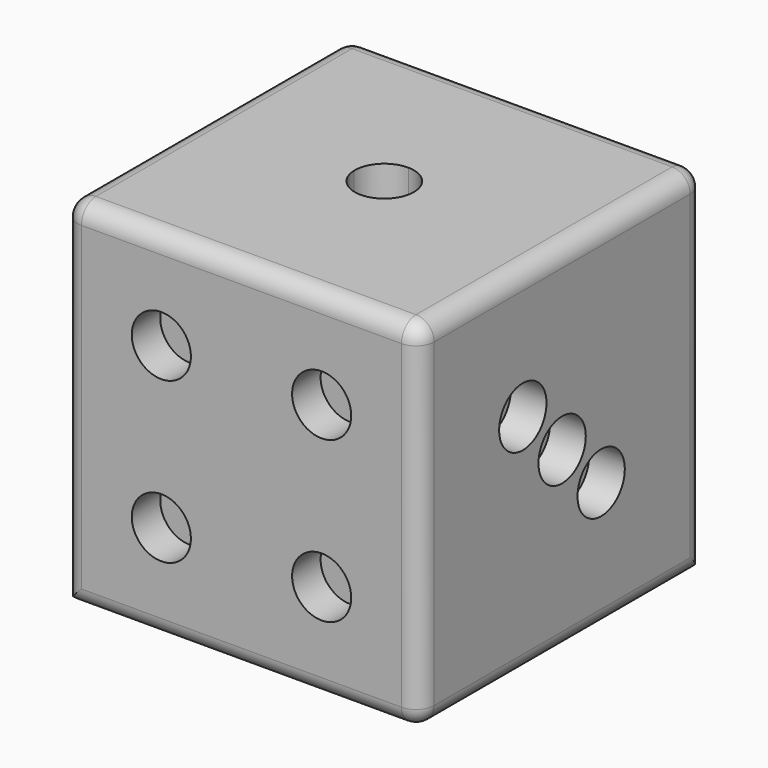
from build123d import *

# Parameters (mm, degrees)
F0_W         = 100
F0_H         = 100
F1_DEPTH     = 100
F2_R         = 5.08
F3_R         = 5.08
F4_T1_DEPTH  = 120.32
F4_T3_DEPTH  = 120.32
F5_T1_DEPTH  = 89.84
F5_S5_W      = 5.08
F5_S5_H      = 5.08
F5_T6_DEPTH  = 5.08
F5_S11_W     = 5.08
F5_S11_H     = 5.08
F5_T12_DEPTH = 5.08
F8_DEPTH     = 10
F10_R        = 8.3
F11_DEPTH    = 10
F12_R        = 8.3
F13_DEPTH    = 10
F9_R         = 8.3
F14_DEPTH    = 10
F15_R        = 8.3
F16_DEPTH    = 10
F17_R        = 8.3
F18_DEPTH    = 10


# Not quite as in the source:
# - a fillet or chamfer that OpenCascade refuses, or shapes differently, is made with other operations: its cross-section is extruded or revolved along the edge and cut away or added


with BuildPart() as f1:
    # F0 (on Top) → F1 (new body)
    with BuildSketch(Plane.XY):
        with Locations((-11.9530703868, 12.5334430486)):
            Rectangle(F0_W, F0_H)
    extrude(amount=F1_DEPTH)

    # F2
    f2_edges = [f1.edges().sort_by_distance(p)[0] for p in [
        (-11.95307, -37.466557, 100),
    ]]
    fillet(f2_edges, radius=F2_R)

    # F3
    f3_edges = [f1.edges().sort_by_distance(p)[0] for p in [
        (-11.95307, -37.466557, 0),
        (38.04693, -37.466557, 47.46),
        (-61.95307, -37.466557, 47.46),
        (-11.95307, 62.533443, 100),
        (-61.95307, 15.073443, 100),
        (38.04693, 15.073443, 100),
        (38.04693, 12.533443, 0),
        (38.04693, 62.533443, 50),
    ]]
    fillet(f3_edges, radius=F3_R)

    # F4: fillet of radius 5.08 on 4 edges, made by hand

    # F4_s2 → F4_t1 (cut)
    with BuildSketch(Plane.YZ.offset(-74.6530703868)):
        with BuildLine():
            ThreePointArc((57.4534430486, 0), (61.045545497, 1.4878975516), (62.5334430486, 5.08))
            Line((62.5334430486, 5.08), (62.5334430486, 0))
            Line((62.5334430486, 0), (57.4534430486, 0))
        make_face()
    extrude(amount=F4_T1_DEPTH, mode=Mode.SUBTRACT)

    # F4_s4 → F4_t3 (cut)
    with BuildSketch(Plane.XZ.offset(-75.2334430486)):
        with BuildLine():
            ThreePointArc((-61.9530703868, 5.08), (-60.4651728352, 1.4878975516), (-56.8730703868, 0))
            Line((-56.8730703868, 0), (-61.9530703868, 0))
            Line((-61.9530703868, 0), (-61.9530703868, 5.08))
        make_face()
    extrude(amount=F4_T3_DEPTH, mode=Mode.SUBTRACT)

    # F5: fillet of radius 5.08 on 1 edges, made by hand

    # F5_s2 → F5_t1 (cut)
    with BuildSketch(Plane.XY.offset(5.08)):
        with BuildLine():
            ThreePointArc((-61.9530703868, 57.4534430486), (-60.4651728352, 61.045545497), (-56.8730703868, 62.5334430486))
            Line((-56.8730703868, 62.5334430486), (-61.9530703868, 62.5334430486))
            Line((-61.9530703868, 62.5334430486), (-61.9530703868, 57.4534430486))
        make_face()
    extrude(amount=F5_T1_DEPTH, mode=Mode.SUBTRACT)


with BuildPart() as f5_tool4:
    # F5_s5 → F5_t6 (new body)
    with BuildSketch(Plane.YZ.offset(-56.8730703868)):
        with Locations((59.9934430486, 2.54)):
            Rectangle(F5_S5_W, F5_S5_H)
    extrude(amount=-F5_T6_DEPTH)

    # F5_s7 → F5_t8 (revolve, cut)
    with BuildSketch(Plane(origin=(-56.8730703868, 57.4534430486, 5.08), x_dir=(0, -0.7071067812, 0.7071067812), z_dir=(0, -0.7071067812, -0.7071067812))):
        with BuildLine():
            ThreePointArc((0, -5.08), (5.08, 0), (0, 5.08))
            Line((0, 5.08), (0, -5.08))
        make_face()
    revolve(axis=Axis((-56.8730703868, 57.4534430486, 5.08), (-1, 0, 0)), mode=Mode.SUBTRACT)


with BuildPart() as f1_1:
    add(f1.part)

    # F5_t3: cut F5_tool4
    add(f5_tool4.part, mode=Mode.SUBTRACT)


with BuildPart() as f5_tool10:
    # F5_s11 → F5_t12 (new body)
    with BuildSketch(Plane.YZ.offset(-56.8730703868)):
        with Locations((59.9934430486, 97.46)):
            Rectangle(F5_S11_W, F5_S11_H)
    extrude(amount=-F5_T12_DEPTH)

    # F5_s13 → F5_t14 (revolve, cut)
    with BuildSketch(Plane(origin=(-56.8730703868, 57.4534430486, 94.92), x_dir=(0, -0.7071067812, -0.7071067812), z_dir=(0, 0.7071067812, -0.7071067812))):
        with BuildLine():
            ThreePointArc((0, -5.08), (5.08, 0), (0, 5.08))
            Line((0, 5.08), (0, -5.08))
        make_face()
    revolve(axis=Axis((-56.8730703868, 57.4534430486, 94.92), (-1, 0, 0)), mode=Mode.SUBTRACT)


with BuildPart() as f1_2:
    add(f1_1.part)

    # F5_t9: cut F5_tool10
    add(f5_tool10.part, mode=Mode.SUBTRACT)

    # F7 (on face) → F8 (cut)
    with BuildSketch(Plane.XY.offset(100)):
        with BuildLine():
            Line((-11.9530703868, 12.5334430486), (-11.9530703868, 21.0658373489))
            ThreePointArc((-11.9530703868, 21.0658373489), (-17.9663578599, 18.5867909487), (-20.3459117026, 12.5334430486))
            Line((-20.3459117026, 12.5334430486), (-11.9530703868, 12.5334430486))
        make_face()
        with BuildLine():
            ThreePointArc((-20.3459117026, 12.5334430486), (-11.932694522, 4.4672112942), (-3.7491813868, 12.7663938329))
            ThreePointArc((-3.7491813868, 12.7663938329), (-6.1463125377, 18.601300803), (-11.9530703868, 21.0658373489))
            Line((-11.9530703868, 21.0658373489), (-11.9530703868, 12.5334430486))
            Line((-11.9530703868, 12.5334430486), (-20.3459117026, 12.5334430486))
        make_face()
    extrude(amount=-F8_DEPTH, mode=Mode.SUBTRACT)

    # F10 (on face) → F11 (cut)
    with BuildSketch(Plane(origin=(0, 62.5334430486, 0), x_dir=(-1, 0, 0), z_dir=(0, 1, 0))):
        with Locations((-10.5468751863, 50)):
            Circle(F10_R)
        with Locations((33.9843742549, 50)):
            Circle(F10_R)
    extrude(amount=-F11_DEPTH, mode=Mode.SUBTRACT)

    # F12 (on face) → F13 (cut)
    with BuildSketch(Plane(origin=(0, 0, 0), x_dir=(1, 0, 0), z_dir=(0, 0, -1))):
        with Locations((-26.988836811, 2.8129873745)):
            Circle(F12_R)
        with Locations((2.9531012963, 2.62785203)):
            Circle(F12_R)
        with Locations((3.9886479591, -28.1644973956)):
            Circle(F12_R)
        with Locations((-27.8392481293, -28.1644973956)):
            Circle(F12_R)
    extrude(amount=-F13_DEPTH, mode=Mode.SUBTRACT)

    # F9 (on face) → F14 (cut)
    with BuildSketch(Plane(origin=(-61.9530703868, 0, 0), x_dir=(0, -1, 0), z_dir=(-1, 0, 0))):
        with Locations((-27.5969797745, 65.0635367259)):
            Circle(F9_R)
        with Locations((-12.5334430486, 50)):
            Circle(F9_R)
        with Locations((2.3449583328, 64.8784013814)):
            Circle(F9_R)
        with Locations((3.3805049956, 34.0860519558)):
            Circle(F9_R)
        with Locations((-28.4473910928, 34.0860519558)):
            Circle(F9_R)
    extrude(amount=-F14_DEPTH, mode=Mode.SUBTRACT)

    # F15 (on face) → F16 (cut)
    with BuildSketch(Plane.YZ.offset(38.0469296132)):
        with Locations((26.2256339981, 36.3078090505)):
            Circle(F15_R)
        with Locations((12.5333450089, 50.0000980397)):
            Circle(F15_R)
        with Locations((-1.261167958, 63.7946110066)):
            Circle(F15_R)
    extrude(amount=-F16_DEPTH, mode=Mode.SUBTRACT)

    # F17 (on face) → F18 (cut)
    with BuildSketch(Plane.XZ.offset(37.4665569514)):
        with Locations((10.5468751863, 27.499999851)):
            Circle(F17_R)
        with Locations((10.5468751863, 72.4999979138)):
            Circle(F17_R)
        with Locations((-34.4531275332, 72.4999979138)):
            Circle(F17_R)
        with Locations((-34.4531275332, 27.499999851)):
            Circle(F17_R)
    extrude(amount=-F18_DEPTH, mode=Mode.SUBTRACT)


solid = f1_2.part
